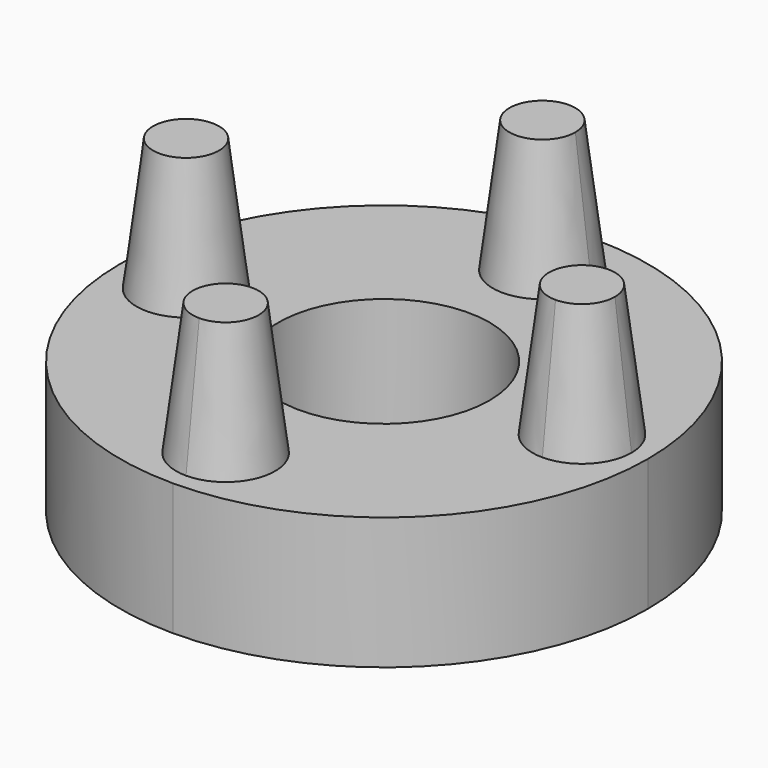
from build123d import *

# Parameters (mm, degrees)
F0_R     = 4
F1_DEPTH = 5
F3_R     = 1.25
F6_COUNT = 4


# Not quite as in the source:
# - a feature names something its author has since deleted; it is built from what else it names


with BuildPart() as f1:
    # F0 (on Top) → F1 (new body)
    with BuildSketch(Plane.XY):
        with BuildLine():
            ThreePointArc((0, 10), (-7.0710678119, -7.0710678119), (10, 0))
            ThreePointArc((10, 0), (7.0710678119, 7.0710678119), (0, 10))
        make_face()
        Circle(F0_R, mode=Mode.SUBTRACT)
        with BuildLine():
            ThreePointArc((2.5, 7.5), (-1.767766953, 5.732233047), (0, 10))
            ThreePointArc((0, 10), (1.767766953, 9.267766953), (2.5, 7.5))
        make_face(mode=Mode.SUBTRACT)
        with BuildLine():
            ThreePointArc((2.5, 7.5), (1.767766953, 9.267766953), (0, 10))
            ThreePointArc((0, 10), (-1.767766953, 5.732233047), (2.5, 7.5))
        make_face()
    extrude(amount=F1_DEPTH)

    # F3 (on offset) → F4 section 0
    with BuildSketch(Plane.XY.offset(10)):
        with Locations((0, 7.5)):
            Circle(F3_R)
    # F0 (on Top) → F4 section 1
    with BuildSketch(Plane.XY):
        with BuildLine():
            ThreePointArc((2.5, 7.5), (1.767766953, 9.267766953), (0, 10))
            ThreePointArc((0, 10), (-1.767766953, 5.732233047), (2.5, 7.5))
        make_face()
    loft()

    # F6: F1 ×4 about axis
    f6_axis = Axis((0, 0, 16.9871691614), (0, 0, 1))


with BuildPart() as f1_1:
    add(f1.part)
    for i in range(1, F6_COUNT):
        add(f1.part.rotate(f6_axis, i * 360 / F6_COUNT))


solid = f1_1.part
